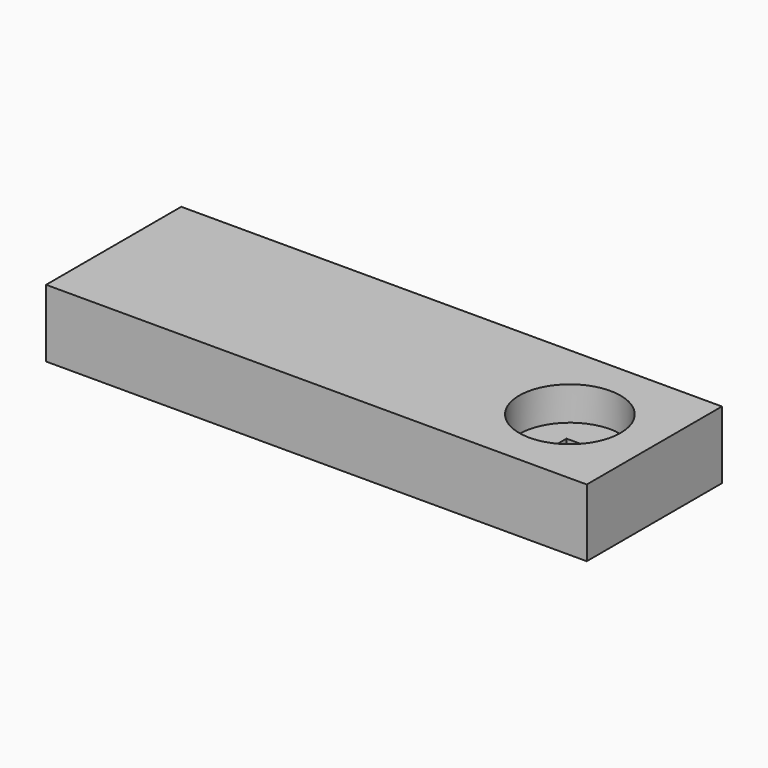
from build123d import *

# Parameters (mm, degrees)
F0_W     = 80
F0_H     = 25
F0_R     = 7.5
F1_DEPTH = 5
F2_W     = 80
F2_H     = 25
F2_R     = 7.5
F2_W_2   = 5
F2_H_2   = 5
F3_DEPTH = 5


with BuildPart() as f1:
    # F0 (on Top) → F1 (new body)
    with BuildSketch(Plane.XY):
        with Locations((-49.0031225234, 12.5)):
            Rectangle(F0_W, F0_H)
        with Locations((-21.5031225234, 12.5)):
            Circle(F0_R, mode=Mode.SUBTRACT)
    extrude(amount=F1_DEPTH)

    # F2 (on face) → F3 (join)
    with BuildSketch(Plane(origin=(0, 0, 0), x_dir=(1, 0, 0), z_dir=(0, 0, -1))):
        with Locations((-49.0031225234, -12.5)):
            Rectangle(F2_W, F2_H)
        with Locations((-21.5031225234, -12.5)):
            Circle(F2_R, mode=Mode.SUBTRACT)
        with Locations((-21.5031225234, -12.5)):
            Circle(F2_R)
        with Locations((-21.5031225234, -12.5)):
            Rectangle(F2_W_2, F2_H_2, mode=Mode.SUBTRACT)
    extrude(amount=F3_DEPTH)


solid = f1.part
